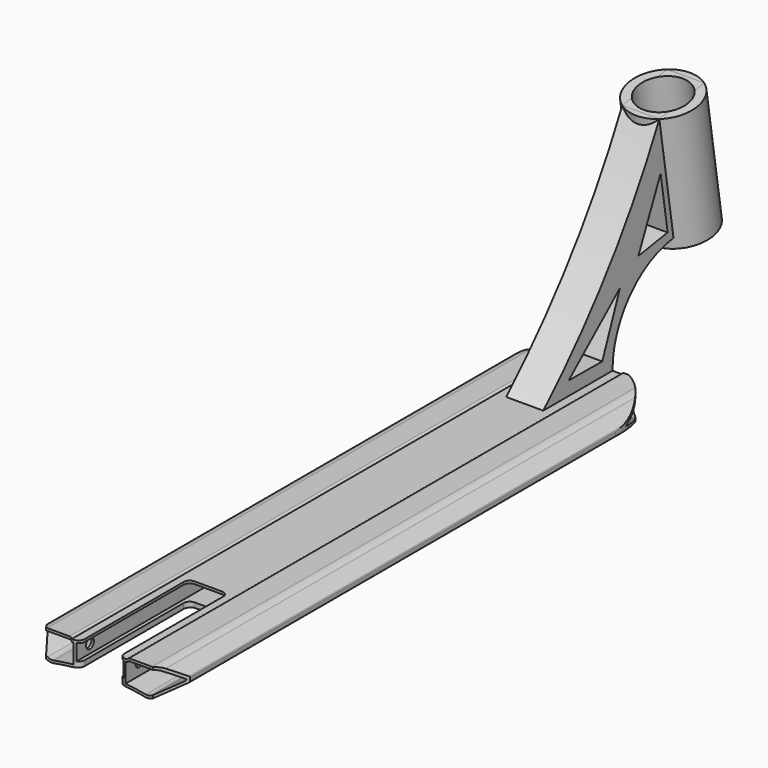
from build123d import *

# Parameters (mm, degrees)
F1_DEPTH       = 250
F2_W           = 38
F2_H           = 13
F3_DEPTH       = 250
F4_T1_DEPTH    = 509.3674969976
F5_R           = 9
F6_R           = 1
F8_DEPTH       = 500.001
F10_DEPTH      = 24.4523840141
F10_DEPTH_BACK = 527
F12_DEPTH      = 527
F12_DEPTH_BACK = 24.4523841141
F13_F1_R       = 4.9999
F13_F2_R       = 4.9999
F13_F3_R       = 5
F13_F4_R       = 5
F13_F5_R       = 5
F13_F6_R       = 5
F15_DEPTH      = 15
F16_R          = 27.4590604355
F17_DEPTH      = 100
F19_D          = 40
F21_D          = 8
F21_DEPTH      = 50
F21_TIP        = 2.4034424761
F23_DEPTH      = 72.5010001


# Not quite as in the source:
# - a fillet or chamfer that OpenCascade refuses, or shapes differently, is made with other operations: its cross-section is extruded or revolved along the edge and cut away or added
# - a fillet or chamfer is up to 0.001 mm smaller than in the source, because OpenCascade refuses the exact size
# - an extrude ends at something that could not be found from the text; its depth is read off the source's solid


with BuildPart() as f1:
    # F0 (on Front) → F1 (new body, symmetric)
    with BuildSketch(Plane.XZ):
        with BuildLine():
            Line((22.5, 23.1513840141), (0, 23.1513840141))
            Line((0, 23.1513840141), (-22.5, 23.1513840141))
            Line((-22.5, 23.1513840141), (-22.5, 24.4513840141))
            Line((-22.5, 24.4513840141), (-45.5824640741, 24.4513840141))
            Line((-45.5824640741, 24.4513840141), (-57.5, 14.4513840141))
            Line((-57.5, 14.4513840141), (-57.5, 10.4513840141))
            Line((-57.5, 10.4513840141), (-40.1794919243, 0.4513840141))
            ThreePointArc((-40.1794919243, 0.4513840141), (0, 4.5289288725), (40.1794919243, 0.4513840141))
            Line((40.1794919243, 0.4513840141), (57.5, 10.4513840141))
            Line((57.5, 10.4513840141), (57.5, 14.4513840141))
            Line((57.5, 14.4513840141), (45.5824640741, 24.4513840141))
            Line((45.5824640741, 24.4513840141), (22.5, 24.4513840141))
            Line((22.5, 24.4513840141), (22.5, 23.1513840141))
        make_face()
    extrude(amount=F1_DEPTH, both=True)

    # F2 (on Front) → F3 (cut, symmetric)
    with BuildSketch(Plane.XZ):
        with Locations((0, 14.6513840141)):
            Rectangle(F2_W, F2_H)
    extrude(amount=F3_DEPTH, both=True, mode=Mode.SUBTRACT)

    # F4: fillet of radius 2 on 2 edges, made by hand

    # F4_s2 → F4_t1 (cut)
    with BuildSketch(Plane.XZ.offset(-254.6837484988)):
        with BuildLine():
            ThreePointArc((-24.3734993995, 24.4513840141), (-23.2333239744, 24.0945516866), (-22.5, 23.1513840141))
            Line((-22.5, 23.1513840141), (-22.5, 24.4513840141))
            Line((-22.5, 24.4513840141), (-24.3734993995, 24.4513840141))
        make_face()
        with BuildLine():
            ThreePointArc((24.3734993995, 24.4513840141), (23.2333239744, 24.0945516866), (22.5, 23.1513840141))
            Line((22.5, 23.1513840141), (22.5, 24.4513840141))
            Line((22.5, 24.4513840141), (24.3734993995, 24.4513840141))
        make_face()
    extrude(amount=F4_T1_DEPTH, mode=Mode.SUBTRACT)

    # F5
    f5_edges = [f1.edges().sort_by_distance(p)[0] for p in [
        (-45.582464, 0, 24.451384),
        (-40.179492, 0, 0.451384),
        (40.179492, 0, 0.451384),
        (45.582464, 0, 24.451384),
    ]]
    fillet(f5_edges, radius=F5_R)

    # F6
    f6_edges = [f1.edges().sort_by_distance(p)[0] for p in [
        (57.5, 0, 14.451384),
        (57.5, 0, 10.451384),
        (-57.5, 0, 10.451384),
        (-57.5, 0, 14.451384),
    ]]
    fillet(f6_edges, radius=F6_R)

    # F7 (on face) → F8 (cut, through all)
    with BuildSketch(Plane.XZ.offset(250)):
        with BuildLine():
            ThreePointArc((-42.1022690923, 3.8709010064), (-39.7790673433, 3.0327059534), (-37.3093701274, 3.0535140017))
            ThreePointArc((-37.3093701274, 3.0535140017), (-29.1789785809, 4.4103617496), (-21, 5.4343792715))
            Line((-21, 5.4343792715), (-21, 21.1513840141))
            Line((-21, 21.1513840141), (-22.5, 21.1513840141))
            ThreePointArc((-22.5, 21.1513840141), (-23.2333239744, 22.0945516866), (-24.3734993995, 22.4513840141))
            Line((-24.3734993995, 22.4513840141), (-42.3067319657, 22.4513840141))
            ThreePointArc((-42.3067319657, 22.4513840141), (-44.7008729689, 22.0292323596), (-46.8062452335, 20.813695116))
            Line((-46.8062452335, 20.813695116), (-55.7563117574, 13.3036975967))
            ThreePointArc((-55.7563117574, 13.3036975967), (-56.1097188459, 12.4504974108), (-55.6135241478, 11.6716277498))
            Line((-55.6135241478, 11.6716277498), (-42.1022690923, 3.8709010064))
        make_face()
        with BuildLine():
            Line((21, 21.1513840141), (21, 5.4343792715))
            ThreePointArc((21, 5.4343792715), (29.1789785809, 4.4103617496), (37.3093701274, 3.0535140017))
            ThreePointArc((37.3093701274, 3.0535140017), (39.7790673433, 3.0327059534), (42.1022690923, 3.8709010064))
            Line((42.1022690923, 3.8709010064), (55.6135241478, 11.6716277498))
            ThreePointArc((55.6135241478, 11.6716277498), (56.1097188459, 12.4504974108), (55.7563117574, 13.3036975967))
            Line((55.7563117574, 13.3036975967), (46.8062452335, 20.813695116))
            ThreePointArc((46.8062452335, 20.813695116), (44.7008729689, 22.0292323596), (42.3067319657, 22.4513840141))
            Line((42.3067319657, 22.4513840141), (24.3734993995, 22.4513840141))
            ThreePointArc((24.3734993995, 22.4513840141), (23.2333239744, 22.0945516866), (22.5, 21.1513840141))
            Line((22.5, 21.1513840141), (21, 21.1513840141))
        make_face()
    extrude(amount=-F8_DEPTH, mode=Mode.SUBTRACT)

    # F9 (on Top) → F10 (cut, two sides)
    with BuildSketch(Plane.XY) as f10_sk:
        with BuildLine():
            ThreePointArc((-57.5, 200), (0, 257.5), (57.5, 200))
            Line((57.5, 200), (57.5, 280))
            Line((57.5, 280), (-57.5, 280))
            Line((-57.5, 280), (-57.5, 200))
        make_face()
    extrude(amount=F10_DEPTH, mode=Mode.SUBTRACT)
    extrude(f10_sk.sketch, amount=-F10_DEPTH_BACK, mode=Mode.SUBTRACT)

    # F11 (on Top) → F12 (cut, two sides)
    with BuildSketch(Plane.XY) as f12_sk:
        Polygon((-43.2975540478, -250), (-68, -216), (-68, -346), (68, -346), (68, -216), (43.2975540478, -250), (16, -250), (16, -140), (-16, -140), (-16, -250), align=None)
    extrude(amount=-F12_DEPTH, mode=Mode.SUBTRACT)
    extrude(f12_sk.sketch, amount=F12_DEPTH_BACK, mode=Mode.SUBTRACT)

    # F13: fillet of radius 5 on 8 edges, made by hand

    # F13_f1 (radius 5 in the source; OpenCascade refuses exactly that, so slightly less here)
    f13_f1_edges = [f1.edges().sort_by_distance(p)[0] for p in [
        (-16, -250, 22.1513840141),
    ]]
    fillet(f13_f1_edges, radius=F13_F1_R)

    # F13_f2 (radius 5 in the source; OpenCascade refuses exactly that, so slightly less here)
    f13_f2_edges = [f1.edges().sort_by_distance(p)[0] for p in [
        (16, -250, 6.0196427984),
    ]]
    fillet(f13_f2_edges, radius=F13_F2_R)

    # F13_f3
    f13_f3_edges = [f1.edges().sort_by_distance(p)[0] for p in [
        (16, -140, 22.1513840141),
    ]]
    fillet(f13_f3_edges, radius=F13_F3_R)

    # F13_f4
    f13_f4_edges = [f1.edges().sort_by_distance(p)[0] for p in [
        (-16, -140, 22.1513840141),
    ]]
    fillet(f13_f4_edges, radius=F13_F4_R)

    # F13_f5
    f13_f5_edges = [f1.edges().sort_by_distance(p)[0] for p in [
        (-16, -140, 6.0196427984),
    ]]
    fillet(f13_f5_edges, radius=F13_F5_R)

    # F13_f6
    f13_f6_edges = [f1.edges().sort_by_distance(p)[0] for p in [
        (16, -140, 6.0196427984),
    ]]
    fillet(f13_f6_edges, radius=F13_F6_R)

    # F14 (on Right) → F15 (join, symmetric)
    with BuildSketch(Plane.YZ):
        with BuildLine():
            ThreePointArc((297.3819995028, 183.1513840141), (245.9666940414, 97.8136618671), (180, 23.1513840141))
            Line((180, 23.1513840141), (250, 23.1513840141))
            ThreePointArc((250, 23.1513840141), (267.6550746197, 69.6272787008), (311.7145367693, 92.6593051387))
            Line((311.7145367693, 92.6593051387), (313.0254460068, 84.3825499546))
            Line((313.0254460068, 84.3825499546), (358.4591096742, 91.5785353465))
            Line((358.4591096742, 91.5785353465), (342.8156631702, 190.347369406))
            Line((342.8156631702, 190.347369406), (297.3819995028, 183.1513840141))
        make_face()
    extrude(amount=F15_DEPTH, both=True)

    # F16 (on face) → F17 (join, through all)
    with BuildSketch(Plane(origin=(0, -21.0209895784, 132.7213047908), x_dir=(1, 0, 0), z_dir=(0, -0.156434465, 0.9876883406))):
        with Locations((0, 345.3719223914)):
            Circle(F16_R)
    extrude(amount=-F17_DEPTH)

    # F19 (through all)
    with Locations(Plane(origin=(0, -21.0209895784, 132.7213047908), x_dir=(1, 0, 0), z_dir=(0, -0.156434465, 0.9876883406))):
        with Locations((0, 345.3719223914)):
            Hole(F19_D / 2)

    # F21 (one way)
    with BuildSketch(Plane.YZ.offset(21)):
        with Locations((-236, 15.4343792715)):
            Circle(F21_D / 2)
    extrude(amount=-F21_DEPTH, mode=Mode.SUBTRACT)
    with Locations(Plane.YZ.offset(21)):
        with Locations((-236, 15.4343792715)):
            with Locations((0, 0, -(F21_DEPTH + F21_TIP / 2))):  # 118° drill point
                Cone(0, F21_D / 2, F21_TIP, mode=Mode.SUBTRACT)

    # F22 (on face) → F23 (cut, through all)
    with BuildSketch(Plane.YZ.offset(15)):
        Polygon((205.6868169308, 34.2114791274), (239.6868169308, 33.9609570801), (257.5687806787, 78.9609570801), align=None)
        Polygon((305.8015852264, 98.9295560122), (298.6742854118, 143.9295560122), (276.1709350086, 94.2365220609), align=None)
    extrude(amount=-F23_DEPTH, mode=Mode.SUBTRACT)


solid = f1.part
